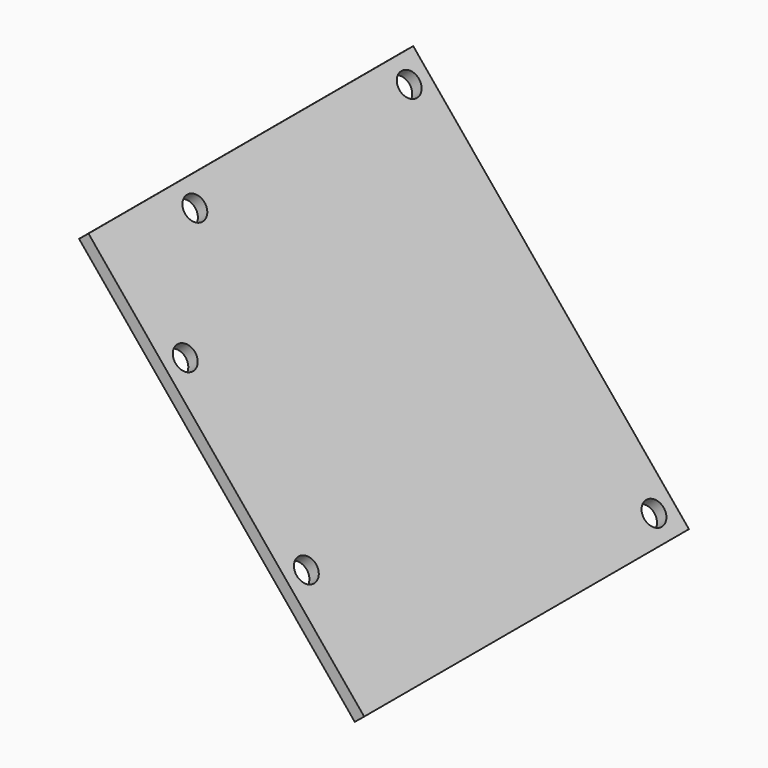
from build123d import *

# Parameters (mm, degrees)
F1_E1_W  = 53.5
F1_E1_H  = 50
F2_DEPTH = 1.5
F3_R     = 1.5
F4_DEPTH = 25


with BuildPart() as f2:
    # F1_E1 (on explicit) → F2 (new body)
    with BuildSketch(Plane(origin=(-36.9205923892, 0, 63.0496794862), x_dir=(0.6347394323, 0, -0.7727262472), z_dir=(0.7727262472, 0, 0.6347394323))):
        with Locations((26.75, 25)):
            Rectangle(F1_E1_W, F1_E1_H)
    extrude(amount=F2_DEPTH)

    # F3 (on face) → F4 (cut)
    with BuildSketch(Plane(origin=(10.0381829655, 0, 8.245650487), x_dir=(0, 1, 0), z_dir=(0.7727262472, 0, 0.6347394323))):
        with Locations((3, 57.1550980691)):
            Circle(F3_R)
        with Locations((3, 33.6550980691)):
            Circle(F3_R)
        with Locations((47, 69.1550980691)):
            Circle(F3_R)
        with Locations((47, 21.6550980691)):
            Circle(F3_R)
        with Locations((14, 69.1550980691)):
            Circle(F3_R)
    extrude(amount=-F4_DEPTH, mode=Mode.SUBTRACT)


solid = f2.part
